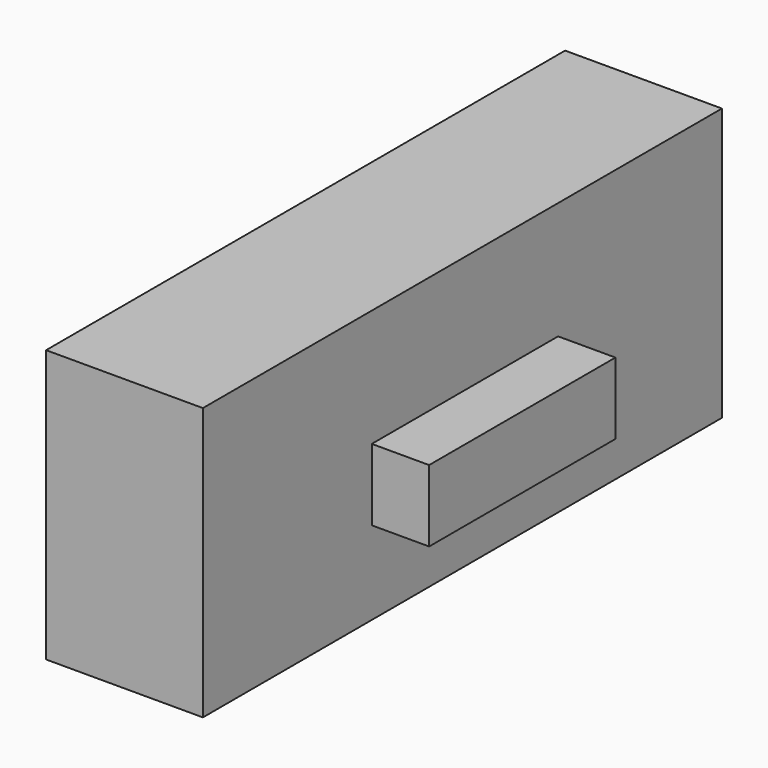
from build123d import *

# Parameters (mm, degrees)
F0_W     = 69.4388896227
F0_H     = 40.5697822571
F1_DEPTH = 181.864
F3_DEPTH = 80.01
F4_DEPTH = 105.41
F5_W     = 103.1131744385
F5_H     = 31.7430943251
F6_DEPTH = 25.4


# Not quite as in the source:
# - the program builds the solid bodies; features that only make, move or delete a surface that nothing else refers to are left out


with BuildPart() as f1:
    # F0 (on Front) → F1 (new body)
    with BuildSketch(Plane.XZ):
        with Locations((34.7194448113, 20.2848911285)):
            Rectangle(F0_W, F0_H)
    extrude(amount=F1_DEPTH)

    # F3 (add): a face of the model
    f3_faces = [f1.faces().sort_by_distance(p)[0] for p in [
        (34.7194448113, -90.932, 40.5697822571),
    ]]
    extrude(f3_faces, amount=F3_DEPTH)

    # F4 (add): a face of the model
    f4_faces = [f1.faces().sort_by_distance(p)[0] for p in [
        (34.7194448113, -181.864, 60.2898911285),
    ]]
    extrude(f4_faces, amount=F4_DEPTH)

    # F5 (on face) → F6 (join)
    with BuildSketch(Plane.YZ.offset(69.4388896227)):
        with Locations((-142.2493308783, 52.7632534504)):
            Rectangle(F5_W, F5_H)
    extrude(amount=F6_DEPTH)


solid = f1.part
